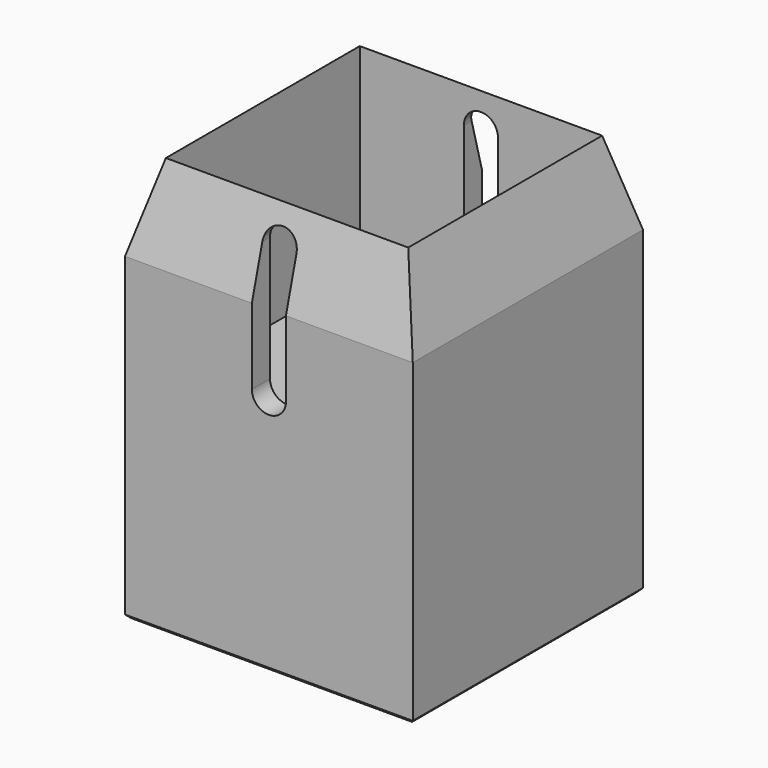
from build123d import *

# Parameters (mm, degrees)
F0_W           = 40.25
F0_H           = 40.25
F1_DEPTH       = 56.45
F2_W           = 33.9
F2_H           = 33.9
F3_DEPTH       = 28
F5_D           = 11
F5_CBORE_D     = 17.25
F5_CBORE_DEPTH = 10
F6_SIZE2       = 11.849251
F6_SIZE        = 3.17499
F8_W           = 4.7625
F8_H           = 17.4625
F9_DEPTH       = 40.251
F10_SIZE       = 0.5


# Not quite as in the source:
# - a fillet or chamfer is up to 0.001 mm smaller than in the source, because OpenCascade refuses the exact size


with BuildPart() as f1:
    # F0 (on Top) → F1 (new body)
    with BuildSketch(Plane.XY):
        Rectangle(F0_W, F0_H)
    extrude(amount=F1_DEPTH)

    # F2 (on face) → F3 (cut)
    with BuildSketch(Plane.XY.offset(56.45)):
        Rectangle(F2_W, F2_H)
    extrude(amount=-F3_DEPTH, mode=Mode.SUBTRACT)

    # F5 (through all)
    with Locations(Plane.XY.offset(28.45)):
        with Locations((0, 0)):
            CounterBoreHole(F5_D / 2, F5_CBORE_D / 2, F5_CBORE_DEPTH)

    # F6 (size 3.175 and 11.849261314 in the source; OpenCascade refuses exactly that, so slightly less here)
    f6_edges = [f1.edges().sort_by_distance(p)[0] for p in [
        (0, 20.125, 56.45),
        (20.125, 0, 56.45),
        (0, -20.125, 56.45),
        (-20.125, 0, 56.45),
    ]]
    f6_side = f1.faces().sort_by_distance((0, -19.555779, 56.45))[0]
    chamfer(f6_edges, length=F6_SIZE, length2=F6_SIZE2, reference=f6_side)

    # F8 (on offset) → F9 (cut, through all)
    with BuildSketch(Plane(origin=(0, 20.125, 0), x_dir=(-1, 0, 0), z_dir=(0, 1, 0))):
        with BuildLine():
            ThreePointArc((-2.38125, 34.00625), (0, 31.625), (2.38125, 34.00625))
            Line((2.38125, 34.00625), (-2.38125, 34.00625))
        make_face()
        with Locations((0, 42.7375)):
            Rectangle(F8_W, F8_H)
        with BuildLine():
            Line((-2.38125, 51.46875), (2.38125, 51.46875))
            ThreePointArc((2.38125, 51.46875), (0, 53.85), (-2.38125, 51.46875))
        make_face()
    extrude(amount=-F9_DEPTH, mode=Mode.SUBTRACT)

    # F10
    f10_edges = [f1.edges().sort_by_distance(p)[0] for p in [
        (20.125, 0, 0),
        (0, -20.125, 0),
        (-20.125, 0, 0),
        (0, 20.125, 0),
    ]]
    chamfer(f10_edges, length=F10_SIZE)


solid = f1.part
